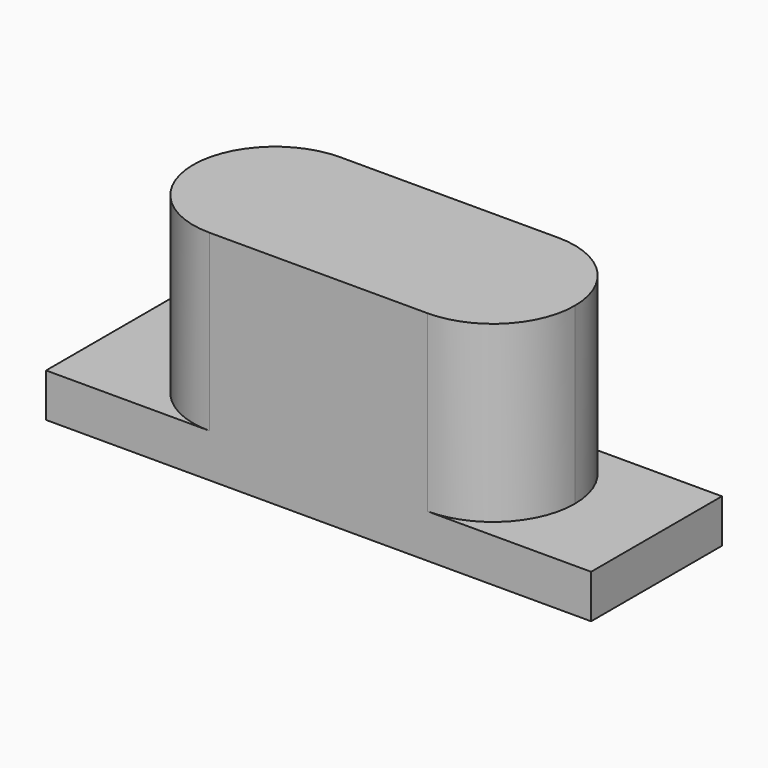
from build123d import *

# Parameters (mm, degrees)
F0_W     = 7
F0_H     = 3
F0_W_2   = 2.5
F0_H_2   = 2.5
F1_DEPTH = 4
F0_W_3   = 1.5
F2_DEPTH = 0.8
F3_R     = 1.49999
F4_DEPTH = 3.6


# Not quite as in the source:
# - a fillet or chamfer is up to 0.001 mm smaller than in the source, because OpenCascade refuses the exact size


with BuildPart() as f1:
    # F0 (on Top) → F1 (new body)
    with BuildSketch(Plane.XY):
        Rectangle(F0_W, F0_H)
        Rectangle(F0_W_2, F0_H_2, mode=Mode.SUBTRACT)
        Rectangle(F0_W_2, F0_H_2)
    extrude(amount=F1_DEPTH)

    # F0 (on Top) → F2 (join)
    with BuildSketch(Plane.XY):
        with Locations((-4.25, 0)):
            Rectangle(F0_W_3, F0_H)
        with Locations((4.25, 0)):
            Rectangle(F0_W_3, F0_H)
    extrude(amount=F2_DEPTH)

    # F3 (radius 1.5 in the source; OpenCascade refuses exactly that, so slightly less here)
    f3_edges = [f1.edges().sort_by_distance(p)[0] for p in [
        (-3.5, 1.5, 2.4),
        (-3.5, -1.5, 2.4),
        (3.5, -1.5, 2.4),
        (3.5, 1.5, 2.4),
    ]]
    fillet(f3_edges, radius=F3_R)

    # F0 (on Top) → F4 (cut)
    with BuildSketch(Plane.XY):
        Rectangle(F0_W_2, F0_H_2)
    extrude(amount=F4_DEPTH, mode=Mode.SUBTRACT)


solid = f1.part
